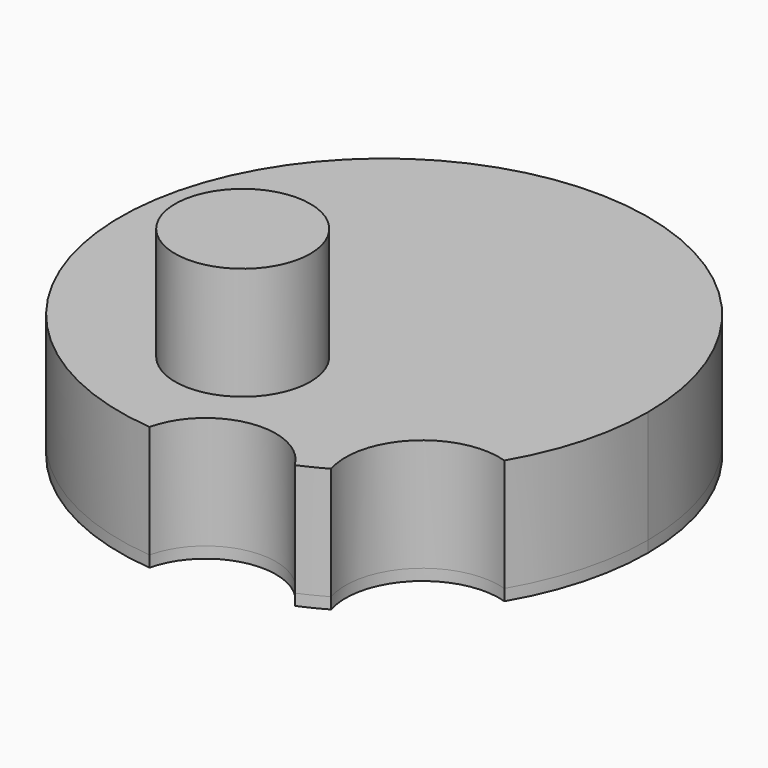
from build123d import *

# Parameters (mm, degrees)
F0_R     = 30
F1_DEPTH = 50
F2_DEPTH = 5
F4_DEPTH = 100


# Not quite as in the source:
# - a feature of the source that left no trace in its solid (it failed there, or was rolled back) is left out


with BuildPart() as f1:
    # F0 (on Top) → F1 (new body)
    with BuildSketch(Plane.XY):
        with BuildLine():
            ThreePointArc((-114.899057503, -52.4928103005), (-106.1762880018, -18.347124739), (-71.9026529407, -10.1414870467))
            ThreePointArc((-71.9026529407, -10.1414870467), (-59.8128831647, 18.5072886108), (-55.6860420642, 49.3274778128))
            ThreePointArc((-55.6860420642, 49.3274778128), (-251.7662613014, 135.8951011853), (-183.6243150436, -67.3241915816))
            ThreePointArc((-183.6243150436, -67.3241915816), (-158.098661689, -43.4558474163), (-126.4336973653, -58.2405309352))
            ThreePointArc((-126.4336973653, -58.2405309352), (-120.5872807659, -55.5254033818), (-114.899057503, -52.4928103005))
        make_face()
        with Locations((-191.2955716252, -6.0283541679)):
            Circle(F0_R, mode=Mode.SUBTRACT)
    extrude(amount=F1_DEPTH)


with BuildPart() as f2:
    # F2 (new): a face of the model
    f2_faces = [f1.part.faces().sort_by_distance(p)[0] for p in [
        (-173.744285094, 57.9244090181, 0),
    ]]
    extrude(f2_faces, amount=F2_DEPTH)


with BuildPart() as f4:
    # F0 (on Top) → F4 (new body)
    with BuildSketch(Plane.XY):
        with Locations((-191.2955716252, -6.0283541679)):
            Circle(F0_R)
    extrude(amount=F4_DEPTH)


solid = Compound([f1.part, f2.part, f4.part])
